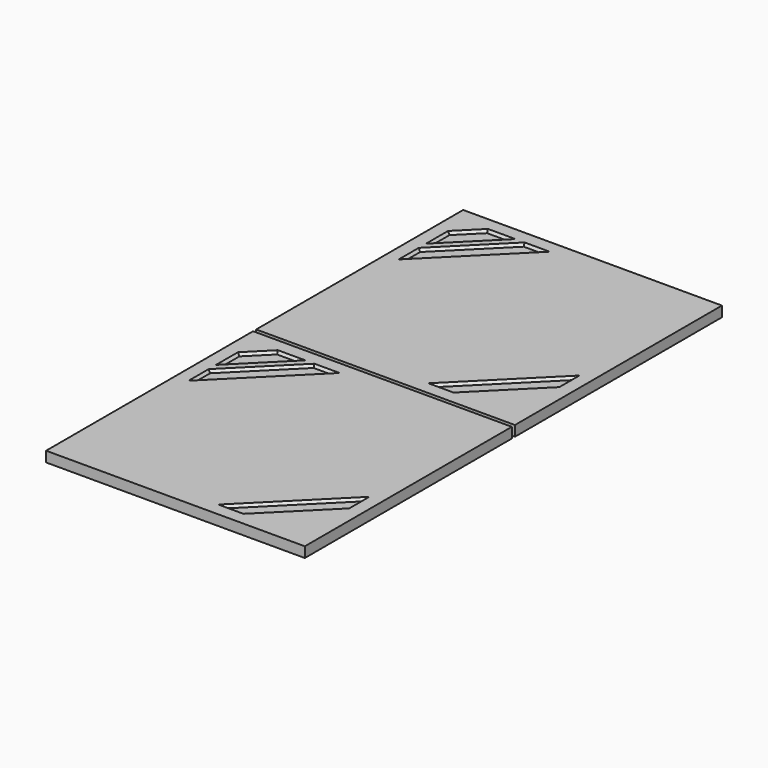
from build123d import *

# Parameters (mm, degrees)
F0_W     = 200
F0_H     = 200
F1_DEPTH = 8
F3_DEPTH = 2
F3_TAPER = 40


# Not quite as in the source:
# - a feature names something its author has since deleted; it is built from what else it names


with BuildPart() as f1:
    # F0 (on Top) → F1 (new body)
    with BuildSketch(Plane.XY):
        Rectangle(F0_W, F0_H)
        Polygon((72.8405151421, -90), (51.6273117065, -90), (90, -51.6273117065), (90, -72.8405151421), align=None, mode=Mode.SUBTRACT)
        Polygon((44.5562379062, -90), (25.1615519314, -90), (90, -25.1615519314), (90, -44.5562379062), align=None, mode=Mode.SUBTRACT)
        Polygon((-90, 25.1615519314), (-90, 44.5562379062), (-44.5562379062, 90), (-25.1615519314, 90), align=None, mode=Mode.SUBTRACT)
        Polygon((-51.6273117065, 90), (-90, 51.6273117065), (-90, 72.8405151421), (-72.8405151421, 90), align=None, mode=Mode.SUBTRACT)
        Polygon((-90, 72.8405151421), (-90, 51.6273117065), (-51.6273117065, 90), (-72.8405151421, 90), align=None)
        Polygon((-44.5562379062, 90), (-90, 44.5562379062), (-90, 25.1615519314), (-25.1615519314, 90), align=None)
        Polygon((90, -25.1615519314), (25.1615519314, -90), (44.5562379062, -90), (90, -44.5562379062), align=None)
        Polygon((90, -51.6273117065), (51.6273117065, -90), (72.8405151421, -90), (90, -72.8405151421), align=None)
    extrude(amount=F1_DEPTH)

    # F2 (on face) → F3 (cut)
    with BuildSketch(Plane.XY.offset(8)):
        Polygon((-90, 51.6273117065), (-51.6273117065, 90), (-72.8405151421, 90), (-90, 72.8405151421), align=None)
        Polygon((-44.5562379062, 90), (-90, 44.5562379062), (-90, 25.1615519314), (-25.1615519314, 90), align=None)
        Polygon((90, -44.5562379062), (90, -25.1615519314), (25.1615519314, -90), (44.5562379062, -90), align=None)
    extrude(amount=-F3_DEPTH, taper=F3_TAPER, mode=Mode.SUBTRACT)


with BuildPart() as f4_1:
    # F4: copy of F1
    add(f1.part.moved(Location((0, 203, 0))))


solid = Compound([f1.part, f4_1.part])
